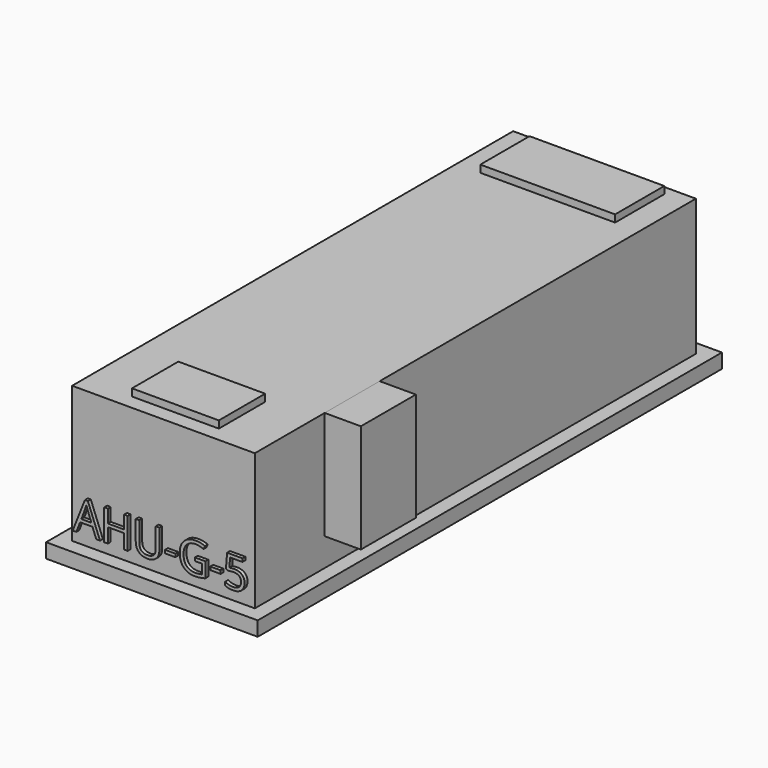
from build123d import *

# Parameters (mm, degrees)
F0_W         = 1282.7
F0_H         = 958.85
F1_DEPTH     = 3870.325
F2_W         = 609.6
F2_H         = 406.4
F3_DEPTH     = 50.8
F4_W         = 1485.9
F4_H         = 101.6
F5_DEPTH     = 101.6
F6_DEPTH     = 3971.925
F7_W         = 482.6
F7_H         = 762
F8_DEPTH     = 254
F9_TEXT_SIZE = 302.8452189432
F10_DEPTH    = 25.4
F11_W        = 946.15
F11_H        = 431.8
F12_DEPTH    = 50.8
F13_W        = 946.15
F13_H        = 431.8
F14_DEPTH    = 50.8


# Not quite as in the source:
# - Text() gives the source's letters only with a copy of the font that has no kerning and outlines rounded to 1/6400 em; it was checked with that copy


with BuildPart() as f1:
    # F0 (on Front) → F1 (new body)
    with BuildSketch(Plane.XZ):
        with Locations((1.4098696411, -73.0132179465)):
            Rectangle(F0_W, F0_H)
    extrude(amount=F1_DEPTH)

    # F2 (on face) → F3 (join)
    with BuildSketch(Plane.XY.offset(406.4117820535)):
        with Locations((1.4098696411, -3562.35)):
            Rectangle(F2_W, F2_H)
    extrude(amount=F3_DEPTH)

    # F9 (on face) → F10 (join)
    with BuildSketch(Plane.XZ.offset(3870.325)):
        with Locations((-615.5583560467, -470.8269834518)):
            Text('AHU-G-5', F9_TEXT_SIZE, font='Open Sans', text_align=(TextAlign.LEFT, TextAlign.BOTTOM))
    extrude(amount=F10_DEPTH)

    # F11 (on face) → F12 (join)
    with BuildSketch(Plane.XY.offset(406.4117820535)):
        with Locations((1.4098696411, -282.575)):
            Rectangle(F11_W, F11_H)
    extrude(amount=F12_DEPTH)

    # F13 (on face) → F14 (join)
    with BuildSketch(Plane(origin=(0, 0, 0), x_dir=(-1, 0, 0), z_dir=(0, 1, 0))):
        with Locations((-1.4098696411, -38.0882179465)):
            Rectangle(F13_W, F13_H)
    extrude(amount=F14_DEPTH)


with BuildPart() as f5:
    # F4 (on face) → F5 (new body)
    with BuildSketch(Plane.XZ.offset(3870.325)):
        with Locations((1.4098696411, -603.2382179465)):
            Rectangle(F4_W, F4_H)
    extrude(amount=F5_DEPTH)

    # F6 (add): a face of the model
    f6_faces = [f5.faces().sort_by_distance(p)[0] for p in [
        (1.4098696411, -3870.325, -603.2382179465),
    ]]
    extrude(f6_faces, amount=F6_DEPTH)


with BuildPart() as f8:
    # F7 (on face) → F8 (new body)
    with BuildSketch(Plane.YZ.offset(642.7598696411)):
        with Locations((-3016.25, 25.4117820535)):
            Rectangle(F7_W, F7_H)
    extrude(amount=F8_DEPTH)


solid = Compound([f1.part, f5.part, f8.part])
